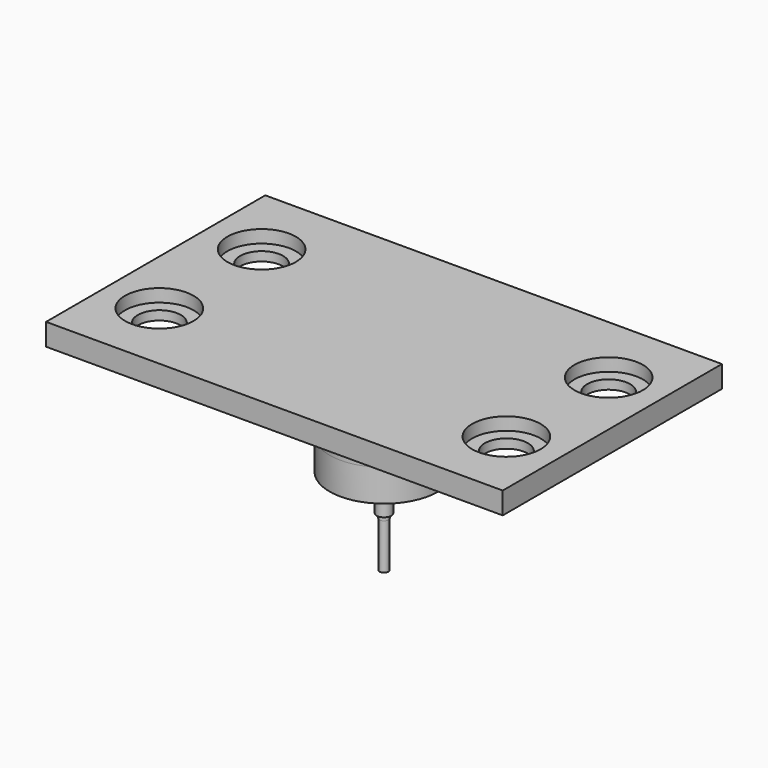
from build123d import *

# Parameters (mm, degrees)
F0_W     = 500
F0_H     = 300
F1_DEPTH = 24
F2_R     = 23.5
F3_DEPTH = 24.001
F2_R_2   = 37.5
F4_DEPTH = 14


# Not quite as in the source:
# - a pattern or mirror of a feature is missing from the dataset's text; its kind, count and spacing are read off the source's solid
# - a feature names something its author has since deleted; it is built from what else it names


with BuildPart() as f1:
    # F0 (on Top) → F1 (new body)
    with BuildSketch(Plane.XY):
        Rectangle(F0_W, F0_H)
    extrude(amount=F1_DEPTH)

    # F2 (on face) → F3 (cut, through all)
    with BuildSketch(Plane.XY.offset(24)):
        with Locations((-190, -70)):
            Circle(F2_R)
    f3 = extrude(amount=-F3_DEPTH, mode=Mode.SUBTRACT)

    # F3_copies: F3 across plane
    add(f3.mirror(Plane(origin=(0, 0, 0), x_dir=(-0.3457053588, 0.9383431168, 0), z_dir=(0.9383431168, 0.3457053588, 0))), mode=Mode.SUBTRACT)

    # F3_copies1: F3 across plane
    add(f3.mirror(Plane(origin=(0, 0, 0), x_dir=(0, 0, 1), z_dir=(1, 0, 0))), mode=Mode.SUBTRACT)

    # F3_copies2: F3 across plane
    add(f3.mirror(Plane.ZX), mode=Mode.SUBTRACT)

    # F2 (on face) → F4 (cut)
    with BuildSketch(Plane.XY.offset(24)):
        with Locations((-190, -70)):
            Circle(F2_R_2)
        with Locations((-190, -70)):
            Circle(F2_R, mode=Mode.SUBTRACT)
    f4 = extrude(amount=-F4_DEPTH, mode=Mode.SUBTRACT)

    # F4_copies: F4 across plane
    add(f4.mirror(Plane(origin=(0, 0, 0), x_dir=(0, 0, 1), z_dir=(1, 0, 0))), mode=Mode.SUBTRACT)

    # F4_copies1: F4 across plane
    add(f4.mirror(Plane.ZX), mode=Mode.SUBTRACT)

    # F4_copies2: F4 across plane
    add(f4.mirror(Plane(origin=(0, 0, 0), x_dir=(-0.3457053588, 0.9383431168, 0), z_dir=(0.9383431168, 0.3457053588, 0))), mode=Mode.SUBTRACT)


with BuildPart() as f6:
    # F5 (on Front) → F6 (revolve)
    with BuildSketch(Plane.XZ):
        Polygon((0, 0), (0, -55), (12, -55), (12, -30), (20, -30), (20, -10), (40, -10), (40, 0), align=None)
    revolve(axis=Axis((0, 0, -27.5), (0, 0, 1)))


with BuildPart() as f7:
    # F5 (on Front) → F7 (revolve)
    with BuildSketch(Plane.XZ):
        Polygon((12, -30), (12, -55), (12, -65), (59.5, -65), (59.5, -30), (20, -30), align=None)
    revolve(axis=Axis((0, 0, -27.5), (0, 0, 1)))


with BuildPart() as f8_1:
    # F8: instance of F7
    add(f7.part.mirror(Plane(origin=(0, 0, -65), x_dir=(1, 0, 0), z_dir=(0, 0, -1))))


with BuildPart() as f9:
    # F5 (on Front) → F9 (revolve)
    with BuildSketch(Plane.XZ):
        Polygon((12, -75), (0, -75), (0, -110), (5, -110), (5, -140), (8, -140), (8, -116.9282032303), (8, -110), (20, -110), (20, -100), (12, -100), align=None)
        Polygon((8, -116.9282032303), (20, -110), (8, -110), align=None)
    revolve(axis=Axis((0, 0, -92.5), (0, 0, 1)))


with BuildPart() as f10:
    # F5 (on Front) → F10 (revolve)
    with BuildSketch(Plane.XZ):
        Polygon((5, -110), (0, -110), (0, -195), (4.75, -195), (4.75, -145), (5, -145), (5, -140), align=None)
    revolve(axis=Axis((0, 0, -152.5), (0, 0, 1)))


solid = Compound([f1.part, f6.part, f7.part, f8_1.part, f9.part, f10.part])
